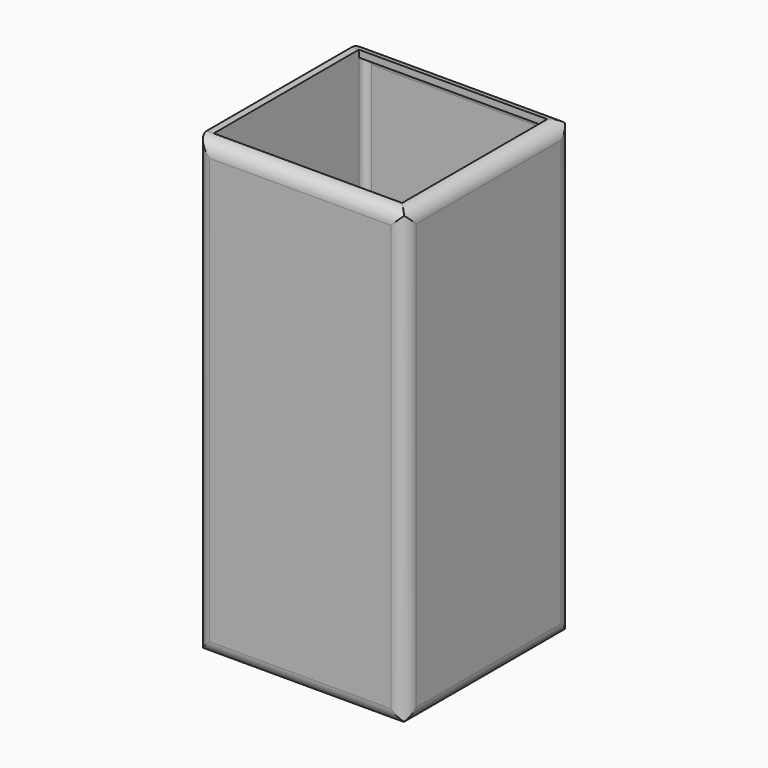
from build123d import *

# Parameters (mm, degrees)
F0_W        = 76.2
F0_H        = 165.1
F1_DEPTH    = 76.2
F2_R        = 5.08
F3_T1_DEPTH = 96.52
F3_T3_DEPTH = 190.5
F4_T1_DEPTH = 96.52
F4_T3_DEPTH = 190.5
F5_T        = 2.54


# Not quite as in the source:
# - a fillet or chamfer that OpenCascade refuses, or shapes differently, is made with other operations: its cross-section is extruded or revolved along the edge and cut away or added
# - a shell that OpenCascade refuses in one call is made with other operations: the cavity is built on its own and cut out


with BuildPart() as f1:
    # F0 (on Right) → F1 (new body)
    with BuildSketch(Plane.YZ):
        Rectangle(F0_W, F0_H)
    extrude(amount=F1_DEPTH)

    # F2
    f2_edges = [f1.edges().sort_by_distance(p)[0] for p in [
        (76.2, 0, 82.55),
        (76.2, -38.1, 0),
        (76.2, 0, -82.55),
        (76.2, 38.1, 0),
    ]]
    fillet(f2_edges, radius=F2_R)

    # F3: fillet of radius 5.08 on 4 edges, made by hand

    # F3_s2 → F3_t1 (cut)
    with BuildSketch(Plane.YZ.offset(-12.7)):
        with BuildLine():
            ThreePointArc((38.1, -77.47), (36.6121024484, -81.0621024484), (33.02, -82.55))
            Line((33.02, -82.55), (38.1, -82.55))
            Line((38.1, -82.55), (38.1, -77.47))
        make_face()
        with BuildLine():
            ThreePointArc((33.02, 82.55), (36.6121024484, 81.0621024484), (38.1, 77.47))
            Line((38.1, 77.47), (38.1, 82.55))
            Line((38.1, 82.55), (33.02, 82.55))
        make_face()
    extrude(amount=F3_T1_DEPTH, mode=Mode.SUBTRACT)

    # F3_s4 → F3_t3 (cut)
    with BuildSketch(Plane.XY.offset(-95.25)):
        with BuildLine():
            ThreePointArc((5.08, 38.1), (1.4878975516, 36.6121024484), (0, 33.02))
            Line((0, 33.02), (0, 38.1))
            Line((0, 38.1), (5.08, 38.1))
        make_face()
    extrude(amount=F3_T3_DEPTH, mode=Mode.SUBTRACT)

    # F4: fillet of radius 5.08 on 4 edges, made by hand

    # F4_s2 → F4_t1 (cut)
    with BuildSketch(Plane.YZ.offset(-12.7)):
        with BuildLine():
            ThreePointArc((-33.02, 82.55), (-36.6121024484, 81.0621024484), (-38.1, 77.47))
            Line((-38.1, 77.47), (-38.1, 82.55))
            Line((-38.1, 82.55), (-33.02, 82.55))
        make_face()
        with BuildLine():
            ThreePointArc((-38.1, -77.47), (-36.6121024484, -81.0621024484), (-33.02, -82.55))
            Line((-33.02, -82.55), (-38.1, -82.55))
            Line((-38.1, -82.55), (-38.1, -77.47))
        make_face()
    extrude(amount=F4_T1_DEPTH, mode=Mode.SUBTRACT)

    # F4_s4 → F4_t3 (cut)
    with BuildSketch(Plane.XY.offset(-95.25)):
        with BuildLine():
            ThreePointArc((0, -33.02), (1.4878975516, -36.6121024484), (5.08, -38.1))
            Line((5.08, -38.1), (0, -38.1))
            Line((0, -38.1), (0, -33.02))
        make_face()
    extrude(amount=F4_T3_DEPTH, mode=Mode.SUBTRACT)

    # F5: shell of thickness 2.54, made by hand


with BuildPart() as f5_core1:
    # F5_t2: copy of F1
    add(f1.part)

    # the walls: a layer under each face that stays
    f5_faces = [f5_core1.faces().sort_by_distance(p)[0] for p in [
        (0, 0, 0),
        (37.3560512242, -36.6121024484, 81.0621024484),
        (74.7121027175, 0, 81.0621021794),
        (37.3560512242, 36.6121024484, 81.0621024484),
        (1.4878975516, -36.6121024484, 0),
        (1.4878975516, 36.6121024484, 0),
        (35.56, 0, -82.55),
        (38.1, -38.1, 0),
        (74.7121027175, -36.6121021794, 0),
        (76.2, 0, 0),
        (74.7121027175, 36.6121021794, 0),
        (38.1, 38.1, 0),
        (37.3560512244, -36.6121024484, -81.0621024484),
        (37.3560512244, 36.6121024484, -81.0621024484),
        (74.7121026774, 0, -81.0621022195),
    ]]
    thicken(f5_faces, amount=-F5_T, mode=Mode.SUBTRACT)


with BuildPart() as f1_1:
    add(f1.part)

    # what is left inside the walls is the cavity
    f5_cavity = [f5_core1.part.solids().sort_by_distance(p)[0] for p in [
        (2.5654, 0, -25.823333),
    ]]
    add(f5_cavity, mode=Mode.SUBTRACT)


solid = f1_1.part
